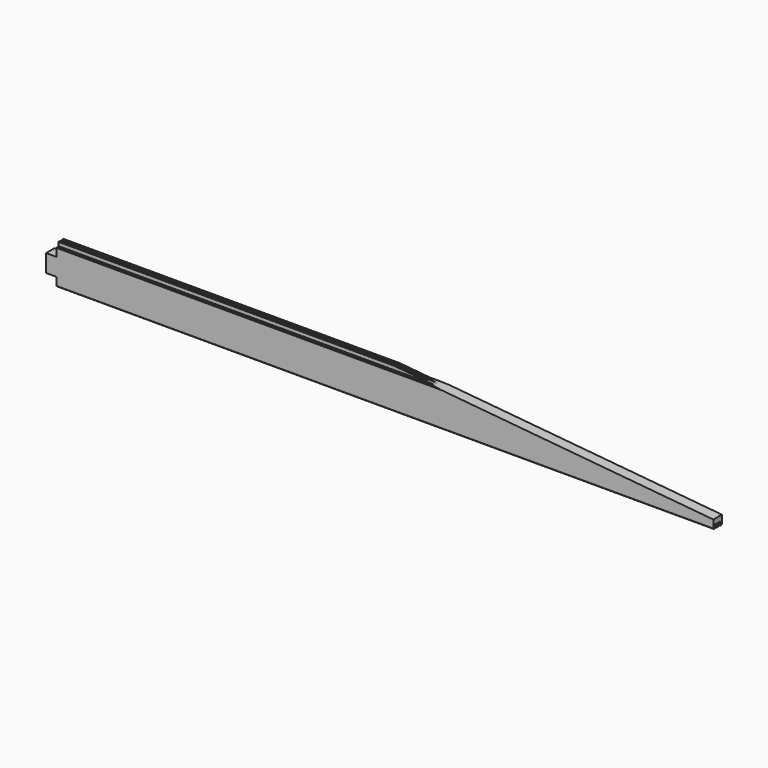
from build123d import *

# Parameters (mm, degrees)
F1_W     = 40
F1_H     = 33
F3_DEPTH = 1275
F2_W     = 80
F2_H     = 100
F4_DEPTH = 25
F6_DEPTH = 25


with BuildPart() as f3:
    # F1 (on Right) → F3 (new body, symmetric)
    with BuildSketch(Plane.YZ):
        Polygon((20, 33), (20, 63), (17, 66), (12, 66), (12, 80), (4, 80), (4, 66), (-4, 66), (-4, 80), (-12, 80), (-12, 66), (-17, 66), (-20, 63), (-20, 33), align=None)
        with Locations((0, 16.5)):
            Rectangle(F1_W, F1_H)
        with Locations((0, -16.5)):
            Rectangle(F1_W, F1_H)
        Polygon((20, -63), (20, -33), (-20, -33), (-20, -63), (-17, -66), (-12, -66), (-12, -52), (-4, -52), (-4, -66), (4, -66), (4, -52), (12, -52), (12, -66), (17, -66), align=None)
    extrude(amount=F3_DEPTH, both=True)

    # F2 (on Front) → F4 (cut, symmetric)
    with BuildSketch(Plane.XZ):
        with Locations((-1275, 83)):
            Rectangle(F2_W, F2_H)
        with Locations((-1275, -83)):
            Rectangle(F2_W, F2_H)
        with Locations((1275, 83)):
            Rectangle(F2_W, F2_H)
        with Locations((1275, -83)):
            Rectangle(F2_W, F2_H)
    extrude(amount=F4_DEPTH, both=True, mode=Mode.SUBTRACT)

    # F5 (on Front) → F6 (cut, symmetric)
    with BuildSketch(Plane.XZ):
        Polygon((1375, 140.368329996), (-616.2874210137, 140.368329996), (1375, -46.110641775), align=None)
    extrude(amount=F6_DEPTH, both=True, mode=Mode.SUBTRACT)


solid = f3.part
